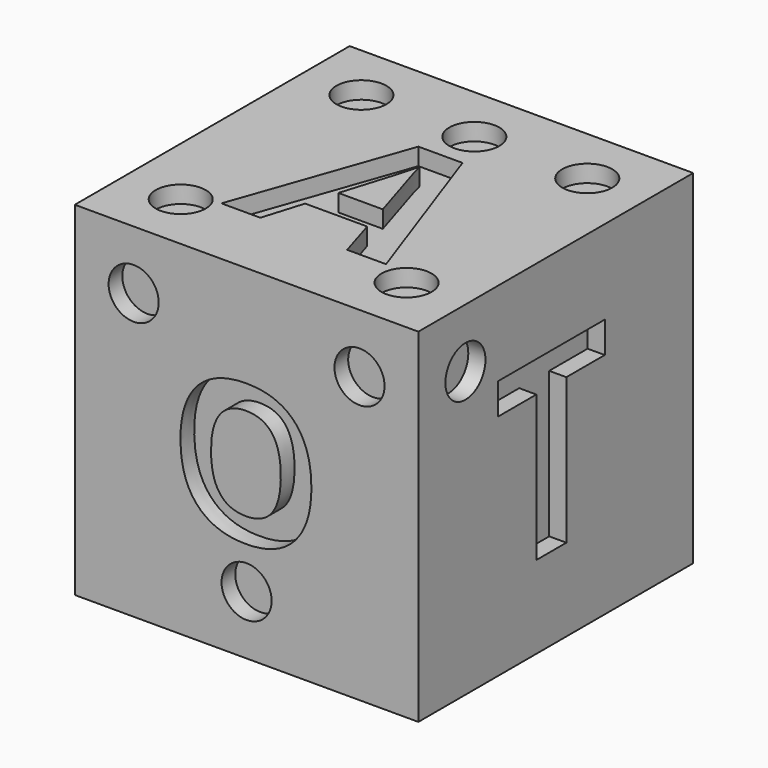
from build123d import *

# Parameters (mm, degrees)
F0_W         = 25.4
F0_H         = 25.4
F1_DEPTH     = 25.4
F2_R         = 1.8512443629
F2_TEXT_SIZE = 18.3200601052
F8_DEPTH     = 1.27
F7_TEXT_SIZE = 19.8405207486
F7_R         = 1.8512443629
F9_DEPTH     = 1.27
F6_R         = 1.8512443629
F6_TEXT_SIZE = 17.6388888889
F10_DEPTH    = 1.27
F3_TEXT_SIZE = 15.4524714829
F3_R         = 1.8512443629
F11_DEPTH    = 1.27
F5_R         = 1.8512443629
F5_TEXT_SIZE = 14.1111111111
F12_DEPTH    = 1.27
F4_TEXT_SIZE = 14.2402180261
F4_R         = 1.8512443629
F13_DEPTH    = 1.27


# Not quite as in the source:
# - Text() gives the source's letters only with a copy of the font that has no kerning and outlines rounded to 1/6400 em; it was checked with that copy


with BuildPart() as f1:
    # F0 (on Top) → F1 (new body)
    with BuildSketch(Plane.XY):
        with Locations((12.7, -12.7)):
            Rectangle(F0_W, F0_H)
    extrude(amount=F1_DEPTH)

    # F2 (on face) → F8 (cut)
    with BuildSketch(Plane.YZ.offset(25.4)):
        with Locations((-21.0487556371, 21.0487556371)):
            Circle(F2_R)
        with Locations((-18.415, 6.1047783621)):
            Text('T', F2_TEXT_SIZE, font='Open Sans', font_style=FontStyle.BOLD, text_align=(TextAlign.LEFT, TextAlign.BOTTOM))
    extrude(amount=-F8_DEPTH, mode=Mode.SUBTRACT)

    # F7 (on face) → F9 (cut)
    with BuildSketch(Plane(origin=(0, 0, 0), x_dir=(-1, 0, 0), z_dir=(0, 1, 0))):
        with Locations((-18.415, 5.5574125305)):
            Text('S', F7_TEXT_SIZE, font='Open Sans', font_style=FontStyle.BOLD, text_align=(TextAlign.LEFT, TextAlign.BOTTOM))
        with Locations((-4.3512443629, 12.7)):
            Circle(F7_R)
        with Locations((-21.0487556371, 12.7)):
            Circle(F7_R)
        with Locations((-21.0487556371, 4.3512443629)):
            Circle(F7_R)
        with Locations((-21.0487556371, 21.0487556371)):
            Circle(F7_R)
        with Locations((-4.3512443629, 21.0487556371)):
            Circle(F7_R)
        with Locations((-4.3512443629, 4.3512443629)):
            Circle(F7_R)
    extrude(amount=-F9_DEPTH, mode=Mode.SUBTRACT)

    # F6 (on face) → F10 (cut)
    with BuildSketch(Plane.XY.offset(25.4)):
        with Locations((21.0487556371, -21.0487556371)):
            Circle(F6_R)
        with Locations((21.0487556371, -4.3512443629)):
            Circle(F6_R)
        with Locations((12.7, -4.3512443629)):
            Circle(F6_R)
        with Locations((4.3512443629, -4.3512443629)):
            Circle(F6_R)
        with Locations((6.5033994772, -19.9785639971)):
            Text('A', F6_TEXT_SIZE, font='Open Sans', font_style=FontStyle.BOLD, text_align=(TextAlign.LEFT, TextAlign.BOTTOM))
        with Locations((4.3512443629, -21.0487556371)):
            Circle(F6_R)
    extrude(amount=-F10_DEPTH, mode=Mode.SUBTRACT)

    # F3 (on face) → F11 (cut)
    with BuildSketch(Plane(origin=(0, 0, 0), x_dir=(1, 0, 0), z_dir=(0, 0, -1))):
        with Locations((6.985, 7.1371102662)):
            Text('H', F3_TEXT_SIZE, font='Open Sans', font_style=FontStyle.BOLD, text_align=(TextAlign.LEFT, TextAlign.BOTTOM))
        with Locations((21.0487556371, 4.3512443629)):
            Circle(F3_R)
        with Locations((4.3512443629, 21.0487556371)):
            Circle(F3_R)
    extrude(amount=-F11_DEPTH, mode=Mode.SUBTRACT)

    # F5 (on face) → F12 (cut)
    with BuildSketch(Plane(origin=(0, 0, 0), x_dir=(0, -1, 0), z_dir=(-1, 0, 0))):
        with Locations((4.3512443629, 4.3512443629)):
            Circle(F5_R)
        with Locations((21.0487556371, 4.3512443629)):
            Circle(F5_R)
        with Locations((4.3512443629, 21.0487556371)):
            Circle(F5_R)
        with Locations((21.0487556371, 21.0487556371)):
            Circle(F5_R)
        with Locations((6.2243229167, 7.62)):
            Text('M', F5_TEXT_SIZE, font='Open Sans', font_style=FontStyle.BOLD, text_align=(TextAlign.LEFT, TextAlign.BOTTOM))
    extrude(amount=-F12_DEPTH, mode=Mode.SUBTRACT)

    # F4 (on face) → F13 (cut)
    with BuildSketch(Plane.XZ.offset(25.4)):
        with Locations((6.985, 7.5735215106)):
            Text('O', F4_TEXT_SIZE, font='Open Sans', font_style=FontStyle.BOLD, text_align=(TextAlign.LEFT, TextAlign.BOTTOM))
        with Locations((12.7, 4.3512443629)):
            Circle(F4_R)
        with Locations((4.3512443629, 21.0487556371)):
            Circle(F4_R)
        with Locations((21.0487556371, 21.0487556371)):
            Circle(F4_R)
    extrude(amount=-F13_DEPTH, mode=Mode.SUBTRACT)


solid = f1.part
